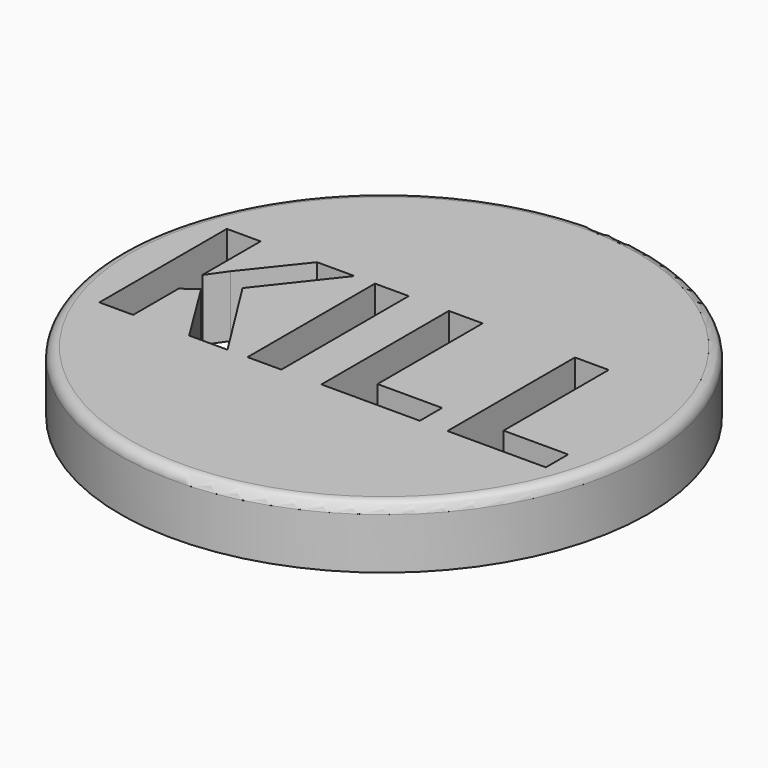
from build123d import *

# Parameters (mm, degrees)
F0_R         = 25.4
F1_DEPTH     = 5.9182
F2_R         = 1
F3_TEXT_SIZE = 21.4709534704
F4_DEPTH     = 25


# Not quite as in the source:
# - Text() gives the source's letters only with a copy of the font that has no kerning and outlines rounded to 1/6400 em; it was checked with that copy


with BuildPart() as f1:
    # F0 (on Top) → F1 (new body)
    with BuildSketch(Plane.XY):
        Circle(F0_R)
    extrude(amount=F1_DEPTH)

    # F2
    f2_edges = [f1.edges().sort_by_distance(p)[0] for p in [
        (-25.4, 0, 5.9182),
    ]]
    fillet(f2_edges, radius=F2_R)

    # F3 (on face) → F4 (cut)
    with BuildSketch(Plane.XY.offset(5.9182)):
        with Locations((-23.1433394556, -7.7295432494)):
            Text('KILL', F3_TEXT_SIZE, font='Open Sans', font_style=FontStyle.BOLD, text_align=(TextAlign.LEFT, TextAlign.BOTTOM))
    extrude(amount=-F4_DEPTH, mode=Mode.SUBTRACT)


solid = f1.part
